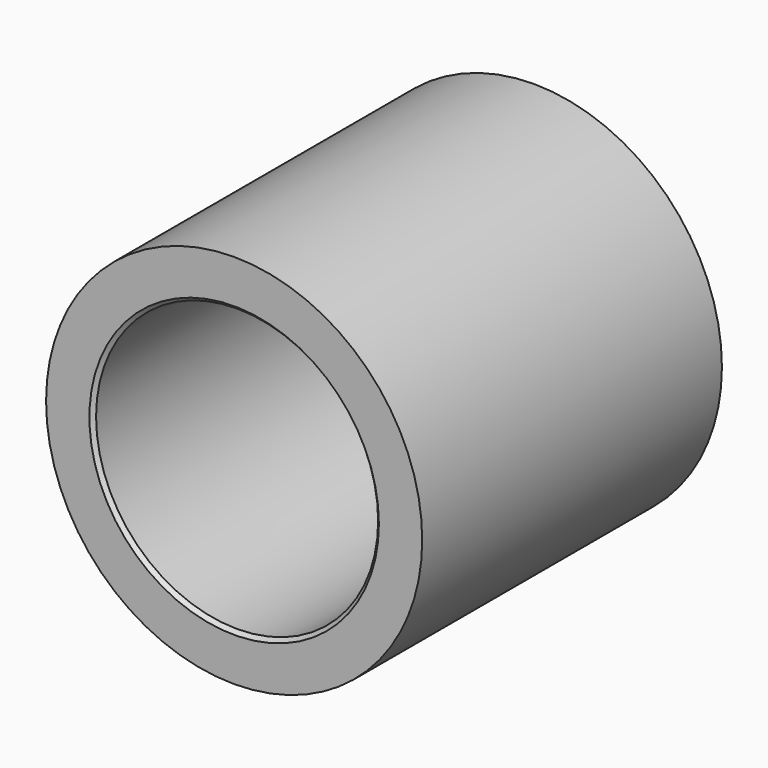
from build123d import *

# Parameters (mm, degrees)
F0_R     = 50.8
F0_R_2   = 38.1
F1_DEPTH = 101.2
F2_R     = 12
F3_SIZE  = 1


with BuildPart() as f1:
    # F0 (on Front) → F1 (new body)
    with BuildSketch(Plane.XZ):
        Circle(F0_R)
        Circle(F0_R_2, mode=Mode.SUBTRACT)
    extrude(amount=F1_DEPTH)

    # F2
    f2_edges = [f1.edges().sort_by_distance(p)[0] for p in [
        (-38.1, 0, 0),
    ]]
    fillet(f2_edges, radius=F2_R)

    # F3
    f3_edges = [f1.edges().sort_by_distance(p)[0] for p in [
        (38.1, -56.6, 0),
        (-38.1, -12, 0),
        (-38.1, -101.2, 0),
    ]]
    chamfer(f3_edges, length=F3_SIZE)


solid = f1.part
